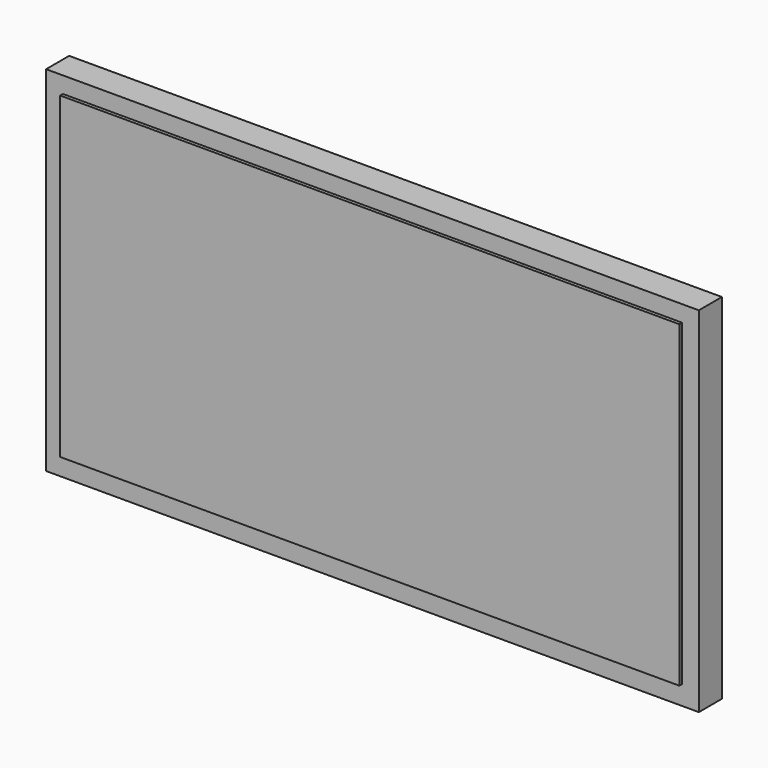
from build123d import *

# Parameters (mm, degrees)
F0_W     = 195.4201161861
F0_H     = 105.9125140309
F1_DEPTH = 8.636
F2_W     = 185.3469088674
F2_H     = 95.2637046576
F3_DEPTH = 1.016
F4_R     = 3.556
F5_DEPTH = 1.016


# Not quite as in the source:
# - a feature names something its author has since deleted; it is built from what else it names


with BuildPart() as f1:
    # F0 (on Front) → F1 (new body)
    with BuildSketch(Plane.XZ):
        with Locations((2.4463534355, -2.8780587018)):
            Rectangle(F0_W, F0_H)
    extrude(amount=F1_DEPTH)

    # F2 (on face) → F3 (join)
    with BuildSketch(Plane.XZ.offset(8.636)):
        with Locations((2.4463497102, -2.4463459849)):
            Rectangle(F2_W, F2_H)
    extrude(amount=F3_DEPTH)

    # F4 (on face) → F5 (join)
    with BuildSketch(Plane(origin=(0, 0, 0), x_dir=(-1, 0, 0), z_dir=(0, 1, 0))):
        with Locations((-74.3977949023, 43.7464751303)):
            Circle(F4_R)
        with Locations((-74.6855959296, -52.2783157172)):
            Circle(F4_R)
        with Locations((74.3977874517, -52.2783157172)):
            Circle(F4_R)
        with Locations((74.9733969569, 43.7464751303)):
            Circle(F4_R)
    extrude(amount=F5_DEPTH)


solid = f1.part
